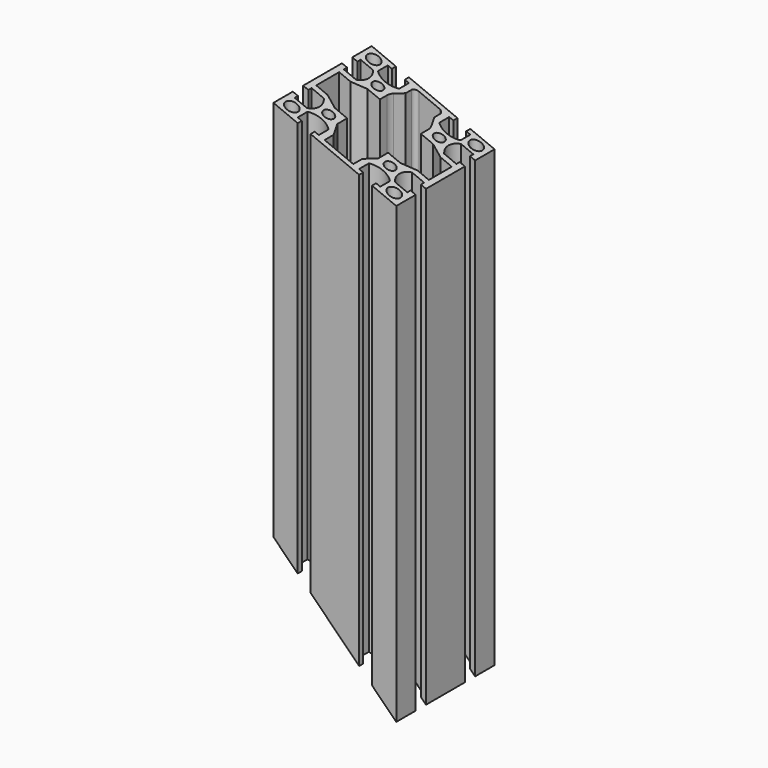
from build123d import *

# Parameters (mm, degrees)
F0_R          = 3
F0_R_2        = 2.5
F1_DEPTH      = 246.7
F2_R          = 2
F3_R          = 7
F6_DEPTH      = 30
F6_DEPTH_BACK = 30


# Not quite as in the source:
# - a feature names something its author has since deleted; it is built from what else it names


with BuildPart() as f1:
    # F0 (on Top) → F1 (new body)
    with BuildSketch(Plane.XY):
        with BuildLine():
            Line((18.15, -30), (30, -30))
            Line((30, -30), (30, -18.15))
            Line((30, -18.15), (27.5, -18.15))
            Line((27.5, -18.15), (27.5, -20.15))
            Line((27.5, -20.15), (21.5477069044, -20.15))
            ThreePointArc((21.5477069044, -20.15), (19.5, -15), (21.5477069044, -9.85))
            Line((21.5477069044, -9.85), (27.5, -9.85))
            Line((27.5, -9.85), (27.5, -11.85))
            Line((27.5, -11.85), (30, -11.85))
            Line((30, -11.85), (30, 11.85))
            Line((30, 11.85), (27.5, 11.85))
            Line((27.5, 11.85), (27.5, 9.85))
            Line((27.5, 9.85), (21.5477069044, 9.85))
            ThreePointArc((21.5477069044, 9.85), (19.5, 15), (21.5477069044, 20.15))
            Line((21.5477069044, 20.15), (27.5, 20.15))
            Line((27.5, 20.15), (27.5, 18.15))
            Line((27.5, 18.15), (30, 18.15))
            Line((30, 18.15), (30, 30))
            Line((30, 30), (18.15, 30))
            Line((18.15, 30), (18.15, 27.5))
            Line((18.15, 27.5), (20.15, 27.5))
            Line((20.15, 27.5), (20.15, 21.5477069044))
            ThreePointArc((20.15, 21.5477069044), (15, 19.5), (9.85, 21.5477069044))
            Line((9.85, 21.5477069044), (9.85, 27.5))
            Line((9.85, 27.5), (11.85, 27.5))
            Line((11.85, 27.5), (11.85, 30))
            Line((11.85, 30), (-11.85, 30))
            Line((-11.85, 30), (-11.85, 27.5))
            Line((-11.85, 27.5), (-9.85, 27.5))
            Line((-9.85, 27.5), (-9.85, 21.5477069044))
            ThreePointArc((-9.85, 21.5477069044), (-15, 19.5), (-20.15, 21.5477069044))
            Line((-20.15, 21.5477069044), (-20.15, 27.5))
            Line((-20.15, 27.5), (-18.15, 27.5))
            Line((-18.15, 27.5), (-18.15, 30))
            Line((-18.15, 30), (-30, 30))
            Line((-30, 30), (-30, 18.15))
            Line((-30, 18.15), (-27.5, 18.15))
            Line((-27.5, 18.15), (-27.5, 20.15))
            Line((-27.5, 20.15), (-21.5477069044, 20.15))
            ThreePointArc((-21.5477069044, 20.15), (-19.5, 15), (-21.5477069044, 9.85))
            Line((-21.5477069044, 9.85), (-27.5, 9.85))
            Line((-27.5, 9.85), (-27.5, 11.85))
            Line((-27.5, 11.85), (-30, 11.85))
            Line((-30, 11.85), (-30, -11.85))
            Line((-30, -11.85), (-27.5, -11.85))
            Line((-27.5, -11.85), (-27.5, -9.85))
            Line((-27.5, -9.85), (-21.5477069044, -9.85))
            ThreePointArc((-21.5477069044, -9.85), (-19.5, -15), (-21.5477069044, -20.15))
            Line((-21.5477069044, -20.15), (-27.5, -20.15))
            Line((-27.5, -20.15), (-27.5, -18.15))
            Line((-27.5, -18.15), (-30, -18.15))
            Line((-30, -18.15), (-30, -30))
            Line((-30, -30), (-18.15, -30))
            Line((-18.15, -30), (-18.15, -27.5))
            Line((-18.15, -27.5), (-20.15, -27.5))
            Line((-20.15, -27.5), (-20.15, -21.5477069044))
            ThreePointArc((-20.15, -21.5477069044), (-15, -19.5), (-9.85, -21.5477069044))
            Line((-9.85, -21.5477069044), (-9.85, -27.5))
            Line((-9.85, -27.5), (-11.85, -27.5))
            Line((-11.85, -27.5), (-11.85, -30))
            Line((-11.85, -30), (11.85, -30))
            Line((11.85, -30), (11.85, -27.5))
            Line((11.85, -27.5), (9.85, -27.5))
            Line((9.85, -27.5), (9.85, -21.5477069044))
            ThreePointArc((9.85, -21.5477069044), (15, -19.5), (20.15, -21.5477069044))
            Line((20.15, -21.5477069044), (20.15, -27.5))
            Line((20.15, -27.5), (18.15, -27.5))
            Line((18.15, -27.5), (18.15, -30))
        make_face()
        with Locations((-25, -25)):
            Circle(F0_R, mode=Mode.SUBTRACT)
        with Locations((-15, -15)):
            Circle(F0_R_2, mode=Mode.SUBTRACT)
        with Locations((25, -25)):
            Circle(F0_R, mode=Mode.SUBTRACT)
        with Locations((15, -15)):
            Circle(F0_R_2, mode=Mode.SUBTRACT)
        with Locations((-25, 25)):
            Circle(F0_R, mode=Mode.SUBTRACT)
        with Locations((-15, 15)):
            Circle(F0_R_2, mode=Mode.SUBTRACT)
        Polygon((-7, 22), (-7, 27.5), (0, 27.5), (7, 27.5), (7, 22), (10, 16), (10, 10), (16, 10), (22, 7), (27.5, 7), (27.5, 0), (27.5, -7), (22, -7), (16, -10), (10, -10), (10, -16), (7, -22), (7, -27.5), (0, -27.5), (-7, -27.5), (-7, -22), (-10, -16), (-10, -10), (-16, -10), (-22, -7), (-27.5, -7), (-27.5, 0), (-27.5, 7), (-22, 7), (-16, 10), (-10, 10), (-10, 16), align=None, mode=Mode.SUBTRACT)
        with Locations((15, 15)):
            Circle(F0_R_2, mode=Mode.SUBTRACT)
        with Locations((25, 25)):
            Circle(F0_R, mode=Mode.SUBTRACT)
    extrude(amount=F1_DEPTH)

    # F2
    f2_edges = [f1.edges().sort_by_distance(p)[0] for p in [
        (-7, 27.5, 123.35),
        (7, 27.5, 123.35),
    ]]
    fillet(f2_edges, radius=F2_R)

    # F3
    f3_edges = [f1.edges().sort_by_distance(p)[0] for p in [
        (-10, 16, 123.35),
        (10, 16, 123.35),
    ]]
    fillet(f3_edges, radius=F3_R)

    # F5 (on Front) → F6 (cut, two sides)
    with BuildSketch(Plane.XZ) as f6_sk:
        Polygon((-21.4844248466, -51.4844248466), (30, 0), (-30.7442165391, 60.7442165391), (-82.2286413857, 9.2597916926), align=None)
        Polygon((69.921577374, 205.311127478), (91.4664718921, 257.3251040235), (-8.4551054819, 298.7139765456), (-30, 246.7), align=None)
    extrude(amount=F6_DEPTH, mode=Mode.SUBTRACT)
    extrude(f6_sk.sketch, amount=-F6_DEPTH_BACK, mode=Mode.SUBTRACT)


solid = f1.part
